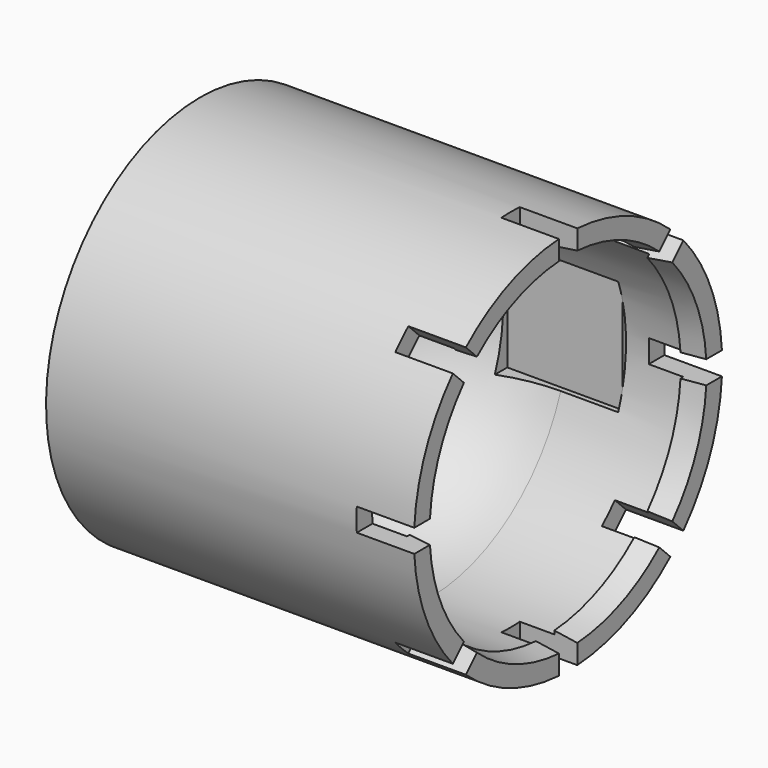
from build123d import *

# Parameters (mm, degrees)
F2_W            = 10
F2_H            = 2
F3_DEPTH        = 16.751
F3_DEPTH_BACK   = 16.751
F3_COPIES_COUNT = 4
F3_COPIES_ANGLE = 135
F4_W            = 10
F4_H            = 10
F5_DEPTH        = 25
F6_W            = 0.65
F6_H            = 10
F7_DEPTH        = 10


# Not quite as in the source:
# - a pattern or mirror of a feature is missing from the dataset's text; its kind, count and spacing are read off the source's solid


with BuildPart() as f1:
    # F0 (on Front) → F1 (revolve)
    with BuildSketch(Plane.XZ):
        with BuildLine():
            Line((0, 15.05), (10, 15.05))
            Line((10, 15.05), (10, 14.75))
            Line((10, 14.75), (12, 15.05))
            Line((12, 15.05), (12, 16.75))
            Line((12, 16.75), (-20, 16.75))
            Line((-20, 16.75), (-20, 9))
            Line((-20, 9), (-12.0624417097, 9))
            ThreePointArc((-12.0624417097, 9), (-6.7473142805, 13.4527413563), (0, 15.05))
        make_face()
    revolve(axis=Axis((10.2357313552, 0, 0), (1, 0, 0)))

    # F2 (on Front) → F3 (cut, two sides)
    with BuildSketch(Plane.XZ) as f3_sk:
        with Locations((12, 0)):
            Rectangle(F2_W, F2_H)
    f3 = extrude(amount=-F3_DEPTH, mode=Mode.SUBTRACT) + extrude(f3_sk.sketch, amount=F3_DEPTH_BACK, mode=Mode.SUBTRACT)

    # F3_copies: F3 ×4 about axis
    f3_copies_axis = Axis((0, 0, 0), (1, 0, 0))
    for i in range(1, F3_COPIES_COUNT):
        add(f3.rotate(f3_copies_axis, i * F3_COPIES_ANGLE / (F3_COPIES_COUNT - 1)), mode=Mode.SUBTRACT)

    # F4 (on Front) → F5 (cut)
    with BuildSketch(Plane.XZ):
        Rectangle(F4_W, F4_H)
    extrude(amount=-F5_DEPTH, mode=Mode.SUBTRACT)

    # F6 (on face) → F7 (join, through all)
    with BuildSketch(Plane.YZ.offset(-5)):
        with Locations((14.9608733114, 0)):
            Rectangle(F6_W, F6_H)
    extrude(amount=F7_DEPTH)


solid = f1.part
